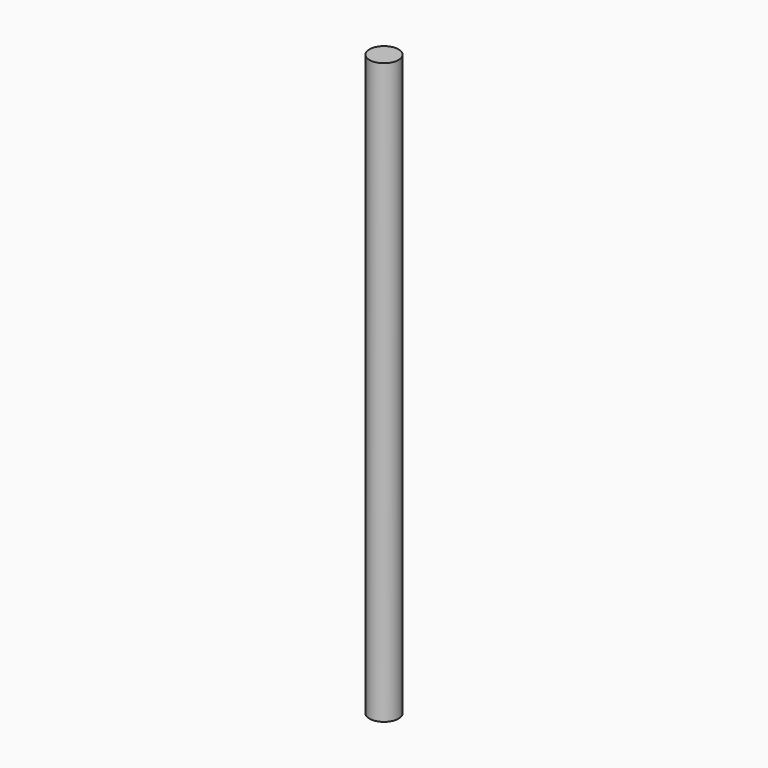
from build123d import *

# Parameters (mm, degrees)
F0_R     = 6.35
F1_DEPTH = 127


# Not quite as in the source:
# - a feature of the source that left no trace in its solid (it failed there, or was rolled back) is left out


with BuildPart() as f1:
    # F0 (on Top) → F1 (new body, symmetric)
    with BuildSketch(Plane.XY):
        Circle(F0_R)
    extrude(amount=F1_DEPTH, both=True)


solid = f1.part
